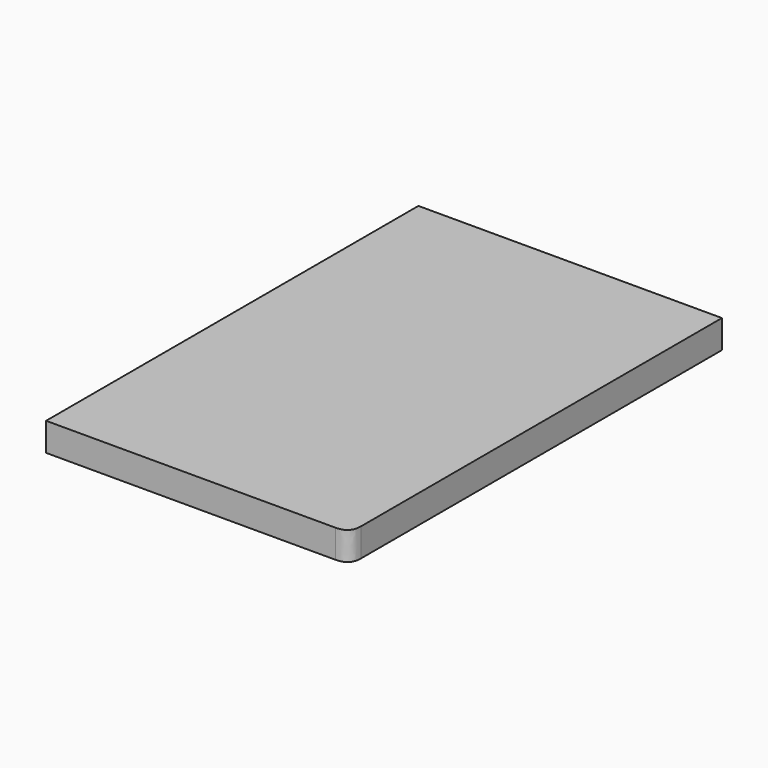
from build123d import *

# Parameters (mm, degrees)
F0_W        = 107.392013073
F0_H        = 164.6451950073
F1_DEPTH    = 10
F2_T1_DEPTH = 35


# Not quite as in the source:
# - a fillet or chamfer that OpenCascade refuses, or shapes differently, is made with other operations: its cross-section is extruded or revolved along the edge and cut away or added


with BuildPart() as f1:
    # F0 (on Top) → F1 (new body)
    with BuildSketch(Plane.XY):
        Rectangle(F0_W, F0_H)
    extrude(amount=F1_DEPTH)

    # F2: fillet of radius 5 on 1 edges, made by hand

    # F2_s2 → F2_t1 (cut)
    with BuildSketch(Plane.XY.offset(-12.5)):
        with BuildLine():
            add(Edge.make_bspline(
                [(48.6960065365, -82.3225975037), (53.6960065365, -82.3225975037), (53.6960065365, -77.3225975037)],
                knots=[0, 0, 0, 1, 1, 1], degree=2, weights=[1, 1, 1]))
            Line((53.6960065365, -77.3225975037), (53.6960065365, -82.3225975037))
            Line((53.6960065365, -82.3225975037), (48.6960065365, -82.3225975037))
        make_face()
    extrude(amount=F2_T1_DEPTH, mode=Mode.SUBTRACT)


solid = f1.part
